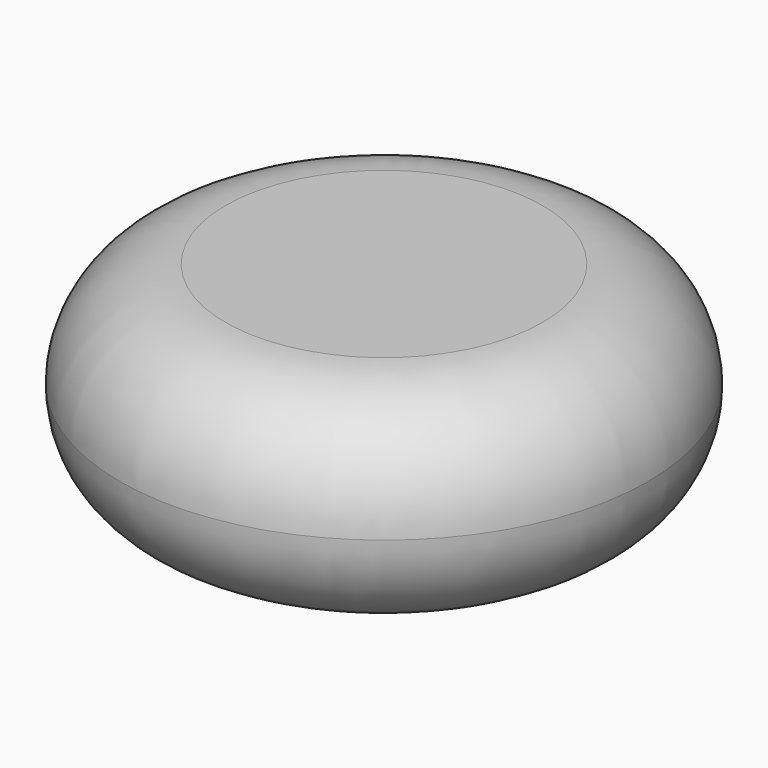
from build123d import *

# Parameters (mm, degrees)
F0_R     = 2.5
F1_DEPTH = 2
F2_R     = 0.99999


# Not quite as in the source:
# - a fillet or chamfer is up to 0.001 mm smaller than in the source, because OpenCascade refuses the exact size


with BuildPart() as f1:
    # F0 (on Top) → F1 (new body)
    with BuildSketch(Plane.XY):
        Circle(F0_R)
    extrude(amount=F1_DEPTH)

    # F2 (radius 1 in the source; OpenCascade refuses exactly that, so slightly less here)
    f2_edges = [f1.edges().sort_by_distance(p)[0] for p in [
        (-2.5, 0, 2),
        (-2.5, 0, 0),
    ]]
    fillet(f2_edges, radius=F2_R)


solid = f1.part
